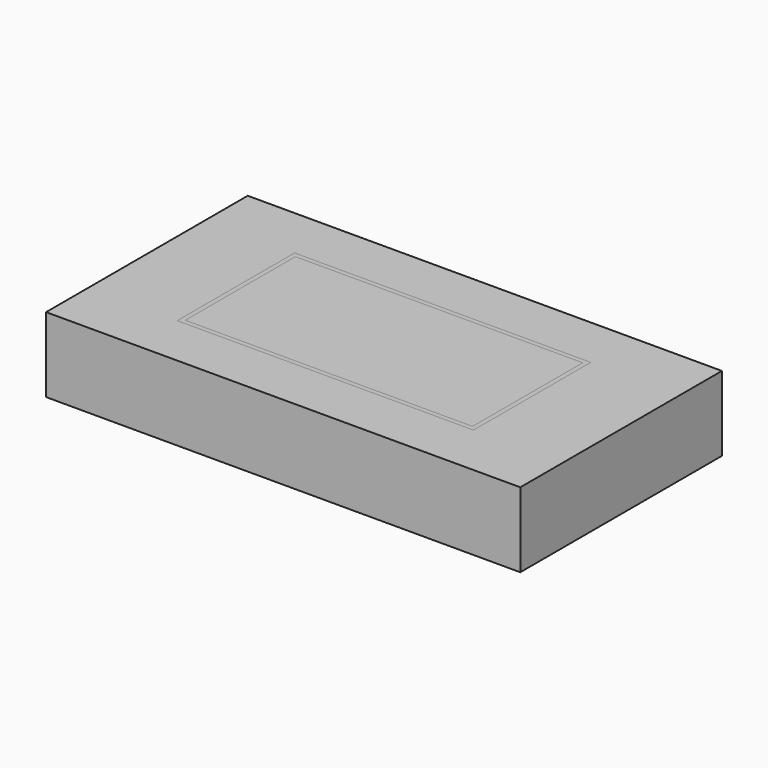
from build123d import *

# Parameters (mm, degrees)
F0_W         = 101.6
F0_H         = 50.8
F1_DEPTH     = 12.7
F2_T         = -2.54
F3_TEXT_SIZE = 8.8194444444
F4_DEPTH     = 6.35
F6_DEPTH     = 3.175
F7_R         = 3.175
F8_DEPTH     = 25.4
F9_SIZE      = 0.508
F10_SIZE     = 0.508
F11_SIZE     = 0.508
F12_W        = 160.9982997179
F12_H        = 85.578083992
F13_DEPTH    = 12.7


# Not quite as in the source:
# - Text() gives the source's letters only with a copy of the font that has no kerning and outlines rounded to 1/6400 em; it was checked with that copy


with BuildPart() as f1:
    # F0 (on Top) → F1 (new body)
    with BuildSketch(Plane.XY):
        Rectangle(F0_W, F0_H)
    extrude(amount=F1_DEPTH)

    # F2
    f2_openings = [f1.faces().sort_by_distance(p)[0] for p in [
        (0, 0, 12.7),
    ]]
    offset(amount=F2_T, openings=f2_openings)

    # F3 (on face) → F4 (join)
    with BuildSketch(Plane.XY.offset(2.54)):
        with Locations((-22.86, 1.1702775188)):
            Text('3 D Printed', F3_TEXT_SIZE, font='Open Sans', font_style=FontStyle.ITALIC, text_align=(TextAlign.LEFT, TextAlign.BOTTOM))
    extrude(amount=F4_DEPTH)

    # F5 (on face) → F6 (join)
    with BuildSketch(Plane(origin=(0, 0, 0), x_dir=(1, 0, 0), z_dir=(0, 0, -1))):
        with BuildLine():
            Line((-50.8, -12.7), (-50.8, 12.7))
            ThreePointArc((-50.8, 12.7), (-63.5, 0), (-50.8, -12.7))
        make_face()
    extrude(amount=-F6_DEPTH)

    # F7 (on face) → F8 (cut)
    with BuildSketch(Plane.XY.offset(3.175)):
        with Locations((-55.88, 0)):
            Circle(F7_R)
    extrude(amount=-F8_DEPTH, mode=Mode.SUBTRACT)

    # F9
    f9_edges = [f1.edges().sort_by_distance(p)[0] for p in [
        (0, -25.4, 0),
        (-50.8, -19.05, 0),
        (50.8, 0, 0),
        (-63.5, 0, 0),
        (0, 25.4, 0),
        (-50.8, 19.05, 0),
        (-59.055, 0, 0),
        (0, -25.4, 12.7),
        (50.8, 0, 12.7),
        (0, 25.4, 12.7),
        (-50.8, 0, 12.7),
        (0, -22.86, 12.7),
        (-48.26, 0, 12.7),
        (0, 22.86, 12.7),
        (48.26, 0, 12.7),
    ]]
    chamfer(f9_edges, length=F9_SIZE)

    # F10
    f10_edges = [f1.edges().sort_by_distance(p)[0] for p in [
        (-63.5, 0, 3.175),
        (-59.055, 0, 3.175),
    ]]
    chamfer(f10_edges, length=F10_SIZE)

    # F11
    f11_edges = [f1.edges().sort_by_distance(p)[0] for p in [
        (-50.8, 25.4, 6.35),
        (50.8, -25.4, 6.35),
        (50.8, 25.4, 6.35),
    ]]
    chamfer(f11_edges, length=F11_SIZE)


with BuildPart() as f13:
    # F12 (on face) → F13 (new body, symmetric)
    with BuildSketch(Plane(origin=(0, 0, 0), x_dir=(1, 0, 0), z_dir=(0, 0, -1))):
        Rectangle(F12_W, F12_H)
    extrude(amount=F13_DEPTH, both=True)

    # F14: cut F1
    add(f1.part, mode=Mode.SUBTRACT)


solid = Compound([f1.part, f13.part])
